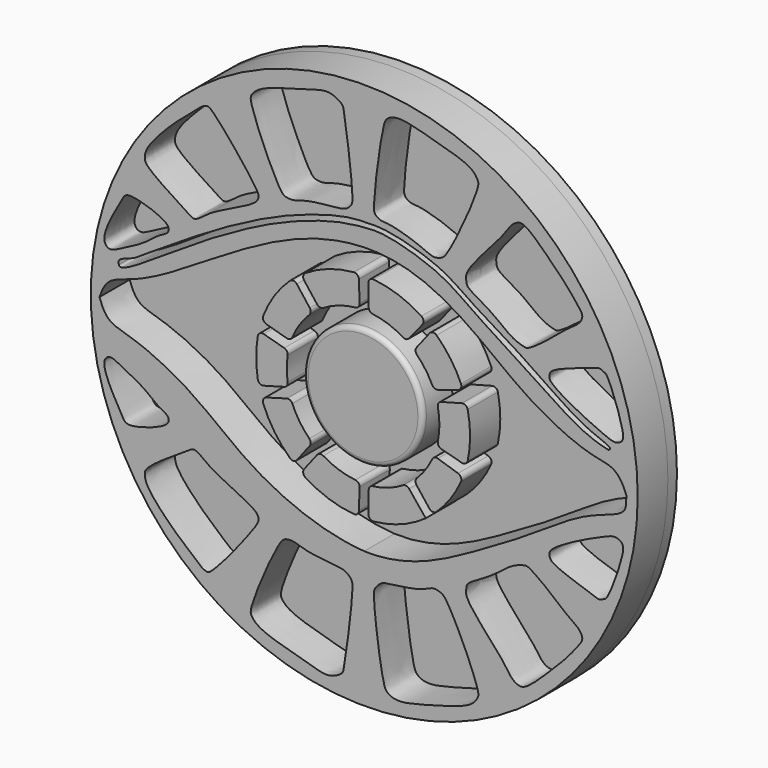
from build123d import *

# Parameters (mm, degrees)
F1_R     = 57.9807392997
F2_DEPTH = 8
F3_DEPTH = 2.4
F0_R     = 12.6313909667
F4_DEPTH = 54
F6_DEPTH = 55
F7_R     = 1


# Not quite as in the source:
# - a feature names something its author has since deleted; it is built from what else it names


with BuildPart() as f2:
    # F1 (on Front) → F2 (new body)
    with BuildSketch(Plane.XZ):
        with Locations((0, -2.0040469244)):
            Circle(F1_R)
    extrude(amount=F2_DEPTH)

    # F0 (on Front) → F4 (cut)
    with BuildSketch(Plane.XZ):
        with BuildLine():
            add(Edge.make_bspline(
                [(-45.8720400929, 29.3476821734), (-44.9458850161, 30.9364265801), (-40.7888769115, 35.3853270873), (-36.7001771058, 38.7900496285), (-34.6197468435, 40.6619407586), (-33.3758440654, 41.2354832358), (-31.9595699175, 40.9055859841), (-22.4143242274, 29.0509154982), (-22.3452683337, 27.6269706045), (-23.0326914864, 25.8895961688), (-32.0132533456, 22.0875896609), (-34.0280106544, 20.310960501), (-36.084758132, 18.9028150512), (-37.5754901046, 20.038678818), (-46.4539772388, 25.5249974668), (-46.5918975329, 27.3951711848), (-46.3485273309, 28.5303067111), (-45.8720400929, 29.3476821734)],
                knots=[0, 0, 0, 0, 0.0968802988, 0.1800402633, 0.2365218543, 0.2733468329, 0.3134327707, 0.4483167787, 0.4887406826, 0.5308655894, 0.6383206338, 0.6999454146, 0.7480177768, 0.7950355756, 0.9063646108, 0.9501571312, 1, 1, 1, 1], degree=3))
        make_face()
        with BuildLine():
            add(Edge.make_bspline(
                [(-22.1556480974, 47.8853674485), (-20.7992304438, 48.6669948913), (-16.5366798433, 49.9829294702), (-12.0003075791, 51.2233677224), (-8.4576541223, 52.261037767), (-6.5459435365, 51.9587387903), (-4.6085321361, 50.884066407), (-4.1576641141, 49.5234420954), (-2.1603987689, 34.0959167095), (-2.6751166911, 32.6279218905), (-3.9511199743, 31.2336907619), (-7.3732540574, 30.9946745905), (-12.4059437506, 30.4742900923), (-14.928228609, 29.390834539), (-16.6657898782, 29.5557437579), (-18.2253273639, 30.3640194535), (-24.4768641225, 44.6327828123), (-23.950725655, 46.432392258), (-22.9828722224, 47.4086845656), (-22.1556480974, 47.8853674485)],
                knots=[0, 0, 0, 0, 0.0757184439, 0.1459001968, 0.2043568265, 0.2476524451, 0.2904860476, 0.3302538222, 0.4525473327, 0.4929515879, 0.5310528746, 0.5886384175, 0.6601040398, 0.711643986, 0.7491960773, 0.7901932344, 0.9121857992, 0.9538223914, 1, 1, 1, 1], degree=3))
        make_face()
        with BuildLine():
            add(Edge.make_bspline(
                [(7.1601802483, 52.0123557998), (8.9376703751, 52.0795646944), (14.3254121397, 50.5132149474), (20.6702791166, 48.8332600235), (23.3119833462, 47.3047450805), (24.0753390093, 45.959476019), (24.6469863359, 44.4964651505), (17.7681529201, 29.5394264711), (16.2119852219, 28.9226346063), (14.5661990197, 28.3362819963), (11.8169563845, 29.9243499614), (5.3757545205, 31.827325229), (3.6867867932, 31.5881828949), (2.1942245815, 32.4284251607), (1.7426767567, 34.2267982143), (3.7226468286, 49.3349834692), (4.7553168681, 51.354629576), (6.1616129993, 51.9745988525), (7.1601802483, 52.0123557998)],
                knots=[0, 0, 0, 0, 0.08687905, 0.1719388515, 0.2262335751, 0.2626983802, 0.3024045396, 0.4317528159, 0.4741506524, 0.5115240134, 0.5694759036, 0.6532547295, 0.695533018, 0.7327117625, 0.7762332962, 0.9019966618, 0.9511926549, 1, 1, 1, 1], degree=3))
        make_face()
        with BuildLine():
            add(Edge.make_bspline(
                [(21.8401215971, 28.0919147535), (22.8519103481, 30.2958755238), (29.7549565997, 37.2984437383), (31.0146896825, 39.9725501338), (32.8146769671, 41.084297997), (34.7094784404, 40.6917258926), (39.6403206901, 35.7904618427), (42.8414303648, 32.5870480881), (45.2962803411, 29.5094222204), (46.5278868565, 27.8955758947), (45.6444092972, 26.0779294117), (43.0190300795, 24.5362156927), (39.824908591, 21.5532601218), (34.9866008861, 18.0365650693), (33.9635306368, 17.989478195), (30.8774724583, 18.927160467), (27.1479792915, 22.5108250015), (21.7037716255, 25.0644592676), (21.6818436938, 26.3827843728), (21.4499972267, 27.2421140348), (21.8401215971, 28.0919147535)],
                knots=[0, 0, 0, 0, 0.1039759174, 0.158365647, 0.1972486804, 0.2362502657, 0.3144628003, 0.3816866846, 0.440396383, 0.4805820433, 0.5191027736, 0.5702430368, 0.6363565766, 0.7080351015, 0.7369611953, 0.7872356927, 0.8591530363, 0.9302518907, 0.9599090825, 1, 1, 1, 1], degree=3))
        make_face()
        with BuildLine():
            add(Edge.make_bspline(
                [(0, 25.6002922521), (9.1488821653, 25.9097882257), (22.3050702942, 18.9112213005), (34.5487227893, 8.1721430016), (47.6598554805, 2.1981379166), (53.2849553554, 2.0400623107), (55.0050297951, -1.0915121178), (55.570102847, -2.5953255458)],
                knots=[0, 0, 0, 0, 0.2811006026, 0.5190104929, 0.7352775741, 0.867921239, 0.9837692807, 0.9837692807, 0.9837692807, 0.9837692807], degree=3))
            add(Edge.make_bspline(
                [(0, 25.6002922521), (-8.7545571515, 25.3269151509), (-22.666236682, 19.2660084957), (-37.4881954946, 9.490203216), (-48.1024089505, 3.5986976032), (-54.4361697427, 2.322260408), (-55.6399523751, -0.5106604776), (-56.1248645625, -1.9204049071)],
                knots=[0, 0, 0, 0, 0.2850018772, 0.5319879097, 0.7337795412, 0.8754593493, 0.9867705847, 0.9867705847, 0.9867705847, 0.9867705847], degree=3))
            add(Edge.make_bspline(
                [(0, -31.0995685501), (-8.5643752903, -30.5085605212), (-23.7247036432, -24.3083001993), (-35.3459880358, -13.5643483696), (-47.8807110218, -7.3557448477), (-54.4103156759, -6.2189282965), (-55.6418100937, -3.3232100999), (-56.1248645625, -1.9204049071)],
                knots=[0, 0, 0, 0, 0.2866139294, 0.5196388602, 0.7332647114, 0.8764431088, 0.9868029126, 0.9868029126, 0.9868029126, 0.9868029126], degree=3))
            add(Edge.make_bspline(
                [(0, -31.0995685501), (9.2587725123, -31.4127819855), (23.0207106869, -23.8444924764), (36.4050417359, -15.9689740109), (47.0537148318, -8.3880302578), (55.944526708, -6.5920219181), (55.4858426223, -3.6826999925), (55.5701028476, -2.5953255457)],
                knots=[0, 0, 0, 0, 0.2844769979, 0.5122610285, 0.7226341191, 0.8831890973, 0.9692841121, 0.9692841121, 0.9692841121, 0.9692841121], degree=3))
        make_face()
        with BuildLine():
            Line((-13.3936041966, -20.7694181827), (-9.4288081106, -15.6364860148))
            ThreePointArc((-9.4288081106, -15.6364860148), (-5.3897281119, -17.6546333764), (-0.9501382805, -18.4775113368))
            Line((-0.9501382805, -18.4775113368), (-1.1691035627, -24.9530745021))
            ThreePointArc((-1.1691035627, -24.9530745021), (-7.5859746616, -23.7513378455), (-13.3936041966, -20.7694181827))
        make_face(mode=Mode.SUBTRACT)
        with BuildLine():
            ThreePointArc((-15.554388985, -7.6924042897), (-13.710559132, -11.3695650493), (-11.0009266455, -14.4645790343))
            Line((-11.0009266455, -14.4645790343), (-14.9205607371, -19.581297758))
            ThreePointArc((-14.9205607371, -19.581297758), (-19.0492242991, -14.9907675612), (-21.7926539835, -9.4597257187))
            Line((-21.7926539835, -9.4597257187), (-15.554388985, -7.6924042897))
        make_face(mode=Mode.SUBTRACT)
        with BuildLine():
            Line((-22.3474123619, 2.7860064816), (-16.0775415554, 1.0612508625))
            ThreePointArc((-16.0775415554, 1.0612508625), (-16.4346932435, -2.319908218), (-16.0775415554, -5.7010672984))
            Line((-16.0775415554, -5.7010672984), (-22.3474123619, -7.4258229175))
            ThreePointArc((-22.3474123619, -7.4258229175), (-22.9296738747, -2.319908218), (-22.3474123619, 2.7860064816))
        make_face(mode=Mode.SUBTRACT)
        with Locations((-0.2513817257, -2.319908218)):
            Circle(F0_R, mode=Mode.SUBTRACT)
        with BuildLine():
            ThreePointArc((0.963872164, -18.4706387465), (5.1409054656, -17.5923074227), (8.943429107, -15.6532645986))
            Line((8.943429107, -15.6532645986), (13.033272033, -20.7188587027))
            ThreePointArc((13.033272033, -20.7188587027), (7.2500148166, -23.7379486126), (0.8468263633, -24.9870064756))
            Line((0.8468263633, -24.9870064756), (0.963872164, -18.4706387465))
        make_face(mode=Mode.SUBTRACT)
        with BuildLine():
            Line((14.4700359172, -19.5057946091), (10.5215810396, -14.4318637404))
            ThreePointArc((10.5215810396, -14.4318637404), (12.9767509972, -11.6886166661), (14.749598787, -8.4621209283))
            Line((14.749598787, -8.4621209283), (20.9349987233, -10.4333174675))
            ThreePointArc((20.9349987233, -10.4333174675), (18.2678592315, -15.3724134246), (14.4700359172, -19.5057946091))
        make_face(mode=Mode.SUBTRACT)
        with BuildLine():
            ThreePointArc((15.3921835453, -6.4645960588), (15.9319297922, -2.319908218), (15.3921835453, 1.8247796228))
            Line((15.3921835453, 1.8247796228), (21.6823376619, 3.5037811846))
            ThreePointArc((21.6823376619, 3.5037811846), (22.4423047186, -2.319908218), (21.6823376619, -8.1435976206))
            Line((21.6823376619, -8.1435976206), (15.3921835453, -6.4645960588))
        make_face(mode=Mode.SUBTRACT)
        with BuildLine():
            Line((-14.945577058, 14.9741378084), (-11.0009266455, 9.8247625984))
            ThreePointArc((-11.0009266455, 9.8247625984), (-13.710559132, 6.7297486134), (-15.554388985, 3.0525878537))
            Line((-15.554388985, 3.0525878537), (-21.7926539835, 4.8199092828))
            ThreePointArc((-21.7926539835, 4.8199092828), (-19.0670498538, 10.3676462084), (-14.945577058, 14.9741378084))
        make_face(mode=Mode.SUBTRACT)
        with BuildLine():
            ThreePointArc((-0.9501382806, 13.8376949009), (-5.389728112, 13.0148169404), (-9.4288081106, 10.9966695788))
            Line((-9.4288081106, 10.9966695788), (-13.3936041966, 16.1296017468))
            ThreePointArc((-13.3936041966, 16.1296017468), (-7.5859746616, 19.1115214096), (-1.1691035627, 20.3132580662))
            Line((-1.1691035627, 20.3132580662), (-0.9501382805, 13.8376949009))
        make_face(mode=Mode.SUBTRACT)
        with BuildLine():
            ThreePointArc((14.749598787, 3.8223044924), (12.9767509972, 7.0488002301), (10.5215810396, 9.7920473045))
            Line((10.5215810396, 9.7920473045), (14.5194335746, 14.929456244))
            ThreePointArc((14.5194335746, 14.929456244), (18.2936119183, 10.7607698454), (20.9215277264, 5.7892080218))
            Line((20.9215277264, 5.7892080218), (14.749598787, 3.8223044924))
        make_face(mode=Mode.SUBTRACT)
        with BuildLine():
            ThreePointArc((8.943429107, 11.0134481627), (5.1409054656, 12.9524909867), (0.963872164, 13.8308223105))
            Line((0.963872164, 13.8308223105), (0.8468263633, 20.3471900397))
            ThreePointArc((0.8468263633, 20.3471900397), (7.2500148166, 19.0981321766), (13.033272033, 16.0790422668))
            Line((13.033272033, 16.0790422668), (8.943429107, 11.0134481627))
        make_face(mode=Mode.SUBTRACT)
        with BuildLine():
            add(Edge.make_bspline(
                [(-52.0109012723, 8.4011282651), (-50.5992949847, 9.1087648175), (-46.7143435763, 10.9848660446), (-43.698233923, 13.7766350176), (-41.5567088579, 14.5433356067), (-41.0076910672, 16.8606926753), (-48.723183894, 19.3083712063), (-50.7538523595, 19.0155136386), (-51.6697883946, 17.2812537672), (-56.2230151191, 9.437567043), (-54.0246766231, 7.3645351228), (-52.8600248112, 7.9754636454), (-52.0109012723, 8.4011282651)],
                knots=[0, 0, 0, 0, 0.1318604735, 0.2440330984, 0.3216920096, 0.386212871, 0.5359397358, 0.6105710387, 0.6857118169, 0.8461214439, 0.9206819686, 1, 1, 1, 1], degree=3))
        make_face()
        with BuildLine():
            add(Edge.make_bspline(
                [(39.8623682559, 15.5091078831), (41.3850114715, 16.7038781044), (48.8462467748, 18.7779833086), (49.6805093788, 19.4144510813), (50.9945172247, 18.8021671256), (51.8020685156, 18.3517424242), (55.4112790828, 8.7493282688), (54.6325140444, 6.9244766151), (53.0592673875, 6.3524969412), (51.1728669181, 7.0362859776), (44.9222620861, 9.802219891), (39.2306573312, 13.2110854926), (39.2750618128, 14.3532978245), (39.2944643217, 15.0634915351), (39.8623682559, 15.5091078831)],
                knots=[0, 0, 0, 0, 0.1502647565, 0.2028546914, 0.254498224, 0.3037728884, 0.4576816743, 0.5230449462, 0.579261749, 0.6452421435, 0.7771021181, 0.9000171252, 0.9439553892, 1, 1, 1, 1], degree=3))
        make_face()
        with BuildLine():
            add(Edge.make_bspline(
                [(39.8623682559, -20.1489243191), (41.3850114715, -21.3436945403), (48.8462467748, -23.4177997445), (49.6805093788, -24.0542675173), (50.9945172247, -23.4419835616), (51.8020685156, -22.9915588602), (55.4112790828, -13.3891447047), (54.6325140444, -11.564293051), (53.0592673875, -10.9923133772), (51.1728669181, -11.6761024135), (44.9222620861, -14.4420363269), (39.2306573312, -17.8509019285), (39.2750618128, -18.9931142604), (39.2944643217, -19.7033079711), (39.8623682559, -20.1489243191)],
                knots=[0, 0, 0, 0, 0.1502647565, 0.2028546914, 0.254498224, 0.3037728884, 0.4576816743, 0.5230449462, 0.579261749, 0.6452421435, 0.7771021181, 0.9000171252, 0.9439553892, 1, 1, 1, 1], degree=3))
        make_face()
        with BuildLine():
            add(Edge.make_bspline(
                [(21.8401215971, -32.7317311894), (22.8519103481, -34.9356919598), (29.7549565997, -41.9382601743), (31.0146896825, -44.6123665698), (32.8146769671, -45.7241144329), (34.7094784404, -45.3315423285), (39.6403206901, -40.4302782787), (42.8414303648, -37.226864524), (45.2962803411, -34.1492386564), (46.5278868565, -32.5353923307), (45.6444092972, -30.7177458477), (43.0190300795, -29.1760321286), (39.824908591, -26.1930765578), (34.9866008861, -22.6763815052), (33.9635306368, -22.629294631), (30.8774724583, -23.5669769029), (27.1479792915, -27.1506414375), (21.7037716255, -29.7042757035), (21.6818436938, -31.0226008087), (21.4499972267, -31.8819304707), (21.8401215971, -32.7317311894)],
                knots=[0, 0, 0, 0, 0.1039759174, 0.158365647, 0.1972486804, 0.2362502657, 0.3144628003, 0.3816866846, 0.440396383, 0.4805820433, 0.5191027736, 0.5702430368, 0.6363565766, 0.7080351015, 0.7369611953, 0.7872356927, 0.8591530363, 0.9302518907, 0.9599090825, 1, 1, 1, 1], degree=3))
        make_face()
        with BuildLine():
            add(Edge.make_bspline(
                [(7.1601802483, -56.6521722358), (8.9380945798, -56.7201025097), (14.32521799, -55.152705443), (20.6703056138, -53.4731093144), (23.3119899805, -51.9445967229), (24.0753123474, -50.5991870333), (24.6472113803, -49.137154652), (17.7660236375, -34.1710039833), (16.2141765935, -33.5709299659), (14.55720833, -32.9413114952), (11.8773267867, -34.8232161421), (5.0847423809, -35.3629672349), (3.5274361871, -35.8372947488), (2.2604814311, -37.1536805726), (1.6869612066, -38.7719261351), (3.7301668532, -53.987580093), (4.7541332046, -55.99243449), (6.1613746874, -56.6140100284), (7.1601802483, -56.6521722358)],
                knots=[0, 0, 0, 0, 0.0867139734, 0.171612155, 0.2258037146, 0.2621992339, 0.3018299487, 0.4309324538, 0.4732497312, 0.5105520801, 0.5683938575, 0.6523858318, 0.6939298034, 0.7332196298, 0.7766584694, 0.9021828753, 0.9512853925, 1, 1, 1, 1], degree=3))
        make_face()
        with BuildLine():
            add(Edge.make_bspline(
                [(-22.1556480974, -52.5251838844), (-20.7992304438, -53.3068113273), (-16.5366798433, -54.6227459061), (-12.0003075791, -55.8631841584), (-8.4576541223, -56.9008542029), (-6.5459435365, -56.5985552263), (-4.6085321361, -55.523882843), (-4.1576641141, -54.1632585313), (-2.1603987689, -38.7357331454), (-2.6751166911, -37.2677383265), (-3.9511199743, -35.8735071978), (-7.3732540574, -35.6344910264), (-12.4059437506, -35.1141065282), (-14.928228609, -34.030650975), (-16.6657898782, -34.1955601938), (-18.2253273639, -35.0038358895), (-24.4768641225, -49.2725992483), (-23.950725655, -51.0722086939), (-22.9828722224, -52.0485010016), (-22.1556480974, -52.5251838844)],
                knots=[0, 0, 0, 0, 0.0757184439, 0.1459001968, 0.2043568265, 0.2476524451, 0.2904860476, 0.3302538222, 0.4525473327, 0.4929515879, 0.5310528746, 0.5886384175, 0.6601040398, 0.711643986, 0.7491960773, 0.7901932344, 0.9121857992, 0.9538223914, 1, 1, 1, 1], degree=3))
        make_face()
        with BuildLine():
            add(Edge.make_bspline(
                [(-45.8720400929, -33.9874986093), (-44.9458850161, -35.576243016), (-40.7888769115, -40.0251435233), (-36.7001771058, -43.4298660645), (-34.6197468435, -45.3017571945), (-33.3758440654, -45.8752996718), (-31.9595699175, -45.54540242), (-22.4143242274, -33.6907319342), (-22.3452683337, -32.2667870404), (-23.0326914864, -30.5294126047), (-32.0132533456, -26.7274060968), (-34.0280106544, -24.9507769369), (-36.084758132, -23.5426314872), (-37.5754901046, -24.6784952539), (-46.4539772388, -30.1648139028), (-46.5918975329, -32.0349876208), (-46.3485273309, -33.1701231471), (-45.8720400929, -33.9874986093)],
                knots=[0, 0, 0, 0, 0.0968802988, 0.1800402633, 0.2365218543, 0.2733468329, 0.3134327707, 0.4483167787, 0.4887406826, 0.5308655894, 0.6383206338, 0.6999454146, 0.7480177768, 0.7950355756, 0.9063646108, 0.9501571312, 1, 1, 1, 1], degree=3))
        make_face()
        with BuildLine():
            add(Edge.make_bspline(
                [(-52.0109012723, -13.0409447011), (-50.5992949847, -13.7485812535), (-46.7143435763, -15.6246824805), (-43.698233923, -18.4164514536), (-41.5567088579, -19.1831520426), (-41.0076910672, -21.5005091112), (-48.723183894, -23.9481876422), (-50.7538523595, -23.6553300746), (-51.6697883946, -21.9210702031), (-56.2230151191, -14.0773834789), (-54.0246766231, -12.0043515587), (-52.8600248112, -12.6152800813), (-52.0109012723, -13.0409447011)],
                knots=[0, 0, 0, 0, 0.1318604735, 0.2440330984, 0.3216920096, 0.386212871, 0.5359397358, 0.6105710387, 0.6857118169, 0.8461214439, 0.9206819686, 1, 1, 1, 1], degree=3))
        make_face()
    extrude(amount=F4_DEPTH, mode=Mode.SUBTRACT)

    # F5 (on Front) → F6 (cut)
    with BuildSketch(Plane.XZ):
        with BuildLine():
            add(Edge.make_bspline(
                [(51.73137784, 4.6237022616), (49.896468826, 5.0776958674), (45.5448231983, 6.3156694638), (33.3893509078, 14.680972585), (22.6044490171, 21.3586639758), (16.207923823, 26.304171434), (4.8009824766, 29.6470981558), (0.0481736613, 29.3899357051), (-6.1422408111, 28.6954137596), (-15.6748216292, 25.5157896337), (-23.7503448112, 21.7356071505), (-34.7509806908, 15.5402445263), (-44.2316332629, 8.9959620913), (-52.0527390458, 4.2837685543), (-52.0109944046, 5.4827621028)],
                knots=[0, 0, 0, 0, 0.067324052, 0.1719605056, 0.269568134, 0.3481140239, 0.4397765124, 0.4990498818, 0.5655665298, 0.6514160853, 0.7336868878, 0.8289535493, 0.9302369652, 1, 1, 1, 1], degree=3))
            add(Edge.make_bspline(
                [(-52.0109944046, 5.4827621028), (-52.0966940247, 5.781693657), (-52.4056832125, 6.554682591), (-49.1220765039, 7.4915860989), (-47.789492815, 8.3688944675), (-34.1606966453, 17.2989965496), (-23.5803151242, 23.0528430066), (-14.768465453, 27.1104420261), (-4.4334143069, 30.2234517257), (0.0294349052, 30.362371512), (5.0255115041, 30.6207139107), (16.592225415, 27.3254613864), (22.5218006476, 22.5720013939), (34.3063868679, 15.955356855), (45.5649678154, 7.5111350234), (51.267454769, 5.7821090955), (52.3764126139, 4.9393260371), (51.9335993716, 4.722615883), (51.73137784, 4.6237022616)],
                knots=[0, 0, 0, 0, 0.0227560624, 0.0647464197, 0.0992039568, 0.197762987, 0.2888149857, 0.3673080298, 0.4487316095, 0.500517777, 0.5559662684, 0.6413110819, 0.7116629501, 0.8038669902, 0.899995487, 0.9591431211, 0.9818095564, 1, 1, 1, 1], degree=3))
        make_face()
    extrude(amount=F6_DEPTH, mode=Mode.SUBTRACT)

    # F7
    f7_edges = [f2.edges().sort_by_distance(p)[0] for p in [
        (-1.169104, -4, 20.313258),
        (-0.950138, -4, 13.837695),
        (-9.428808, -4, 10.99667),
        (-13.393604, -4, 16.129602),
        (-11.000927, -4, 9.824763),
        (-14.945577, -4, 14.974138),
        (-16.077542, -4, 1.061251),
        (-22.347412, -4, 2.786006),
        (-21.792654, -4, 4.819909),
        (-22.347412, -4, -7.425823),
        (-16.077542, -4, -5.701067),
        (-21.792654, -4, -9.459726),
        (-14.920561, -4, -19.581298),
        (-13.393604, -4, -20.769418),
        (-1.169104, -4, -24.953075),
        (0.846826, -4, -24.987006),
        (14.470036, -4, -19.505795),
        (10.521581, -4, -14.431864),
        (15.392184, -4, -6.464596),
        (14.749599, -4, -8.462121),
        (21.682338, -4, -8.143598),
        (15.392184, -4, 1.82478),
        (14.749599, -4, 3.822304),
        (10.521581, -4, 9.792047),
        (8.943429, -4, 11.013448),
        (0.963872, -4, 13.830822),
        (-15.554389, -4, 3.052588),
        (20.921528, -4, 5.789208),
        (14.519434, -4, 14.929456),
        (-0.950138, -4, -18.477511),
        (-9.428808, -4, -15.636486),
        (-11.000927, -4, -14.464579),
        (-15.554389, -4, -7.692404),
        (21.682338, -4, 3.503781),
        (20.934999, -4, -10.433317),
        (0.846826, -4, 20.34719),
        (13.033272, -4, 16.079042),
        (0.963872, -4, -18.470639),
        (8.943429, -4, -15.653265),
        (-12.882773, -8, -2.319908),
    ]]
    fillet(f7_edges, radius=F7_R)


with BuildPart() as f3:
    # F1 (on Front) → F3 (new body)
    with BuildSketch(Plane.XZ):
        with Locations((0, -2.0040469244)):
            Circle(F1_R)
    extrude(amount=-F3_DEPTH)


solid = Compound([f2.part, f3.part])
